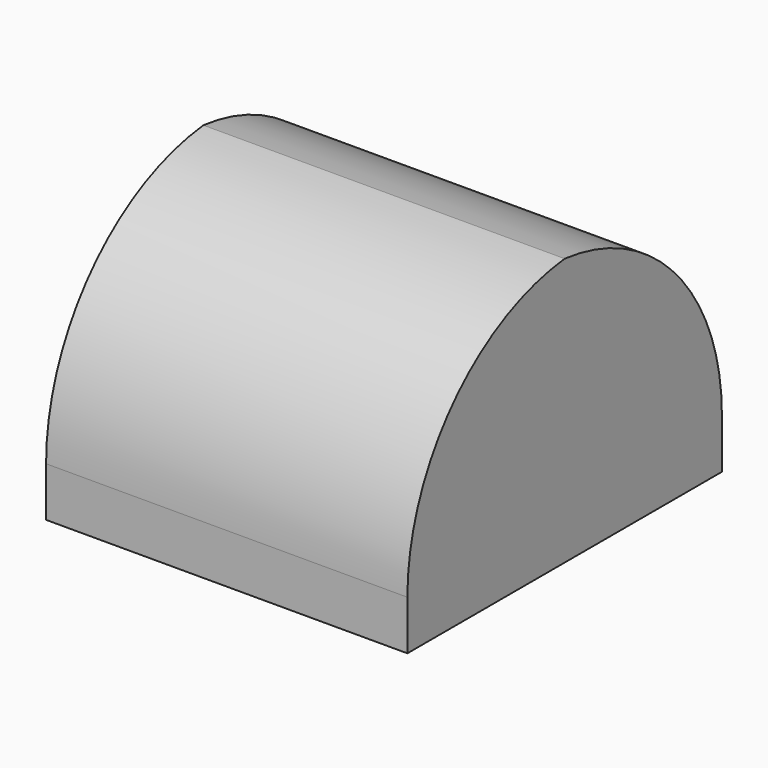
from build123d import *

# Parameters (mm, degrees)
F0_W        = 83.7067794055
F0_H        = 45.5432236195
F1_DEPTH    = 61.976
F2_T1_DEPTH = 336.3431931548
F3_T        = -12.7


# Not quite as in the source:
# - a fillet or chamfer that OpenCascade refuses, or shapes differently, is made with other operations: its cross-section is extruded or revolved along the edge and cut away or added


with BuildPart() as f1:
    # F0 (on Top) → F1 (new body)
    with BuildSketch(Plane.XY):
        with Locations((11.8514457718, -7.8249704093)):
            Rectangle(F0_W, F0_H)
    extrude(amount=F1_DEPTH)

    # F2: fillet of radius 50.8 on 1 edges, made by hand

    # F2_s2 → F2_t1 (cut)
    with BuildSketch(Plane.YZ.offset(-156.3201508057)):
        with BuildLine():
            ThreePointArc((-30.596582219, 11.4487172501), (-17.5304147843, 45.4604487546), (14.9466414005, 61.976))
            Line((14.9466414005, 61.976), (-30.596582219, 61.976))
            Line((-30.596582219, 61.976), (-30.596582219, 11.4487172501))
        make_face()
    extrude(amount=F2_T1_DEPTH, mode=Mode.SUBTRACT)

    # F3
    f3_openings = [f1.faces().sort_by_distance(p)[0] for p in [
        (11.851446, 14.946641, 30.988),
        (11.851446, -7.82497, 0),
    ]]
    offset(amount=F3_T, openings=f3_openings)

    # F4: F1 across face


with BuildPart() as f1_1:
    add(f1.part)
    add(f1.part.mirror(Plane(origin=(11.8514457718, 14.9466414005, 38.893861799), x_dir=(-1, 0, 0), z_dir=(0, 1, 0))))


solid = f1_1.part
